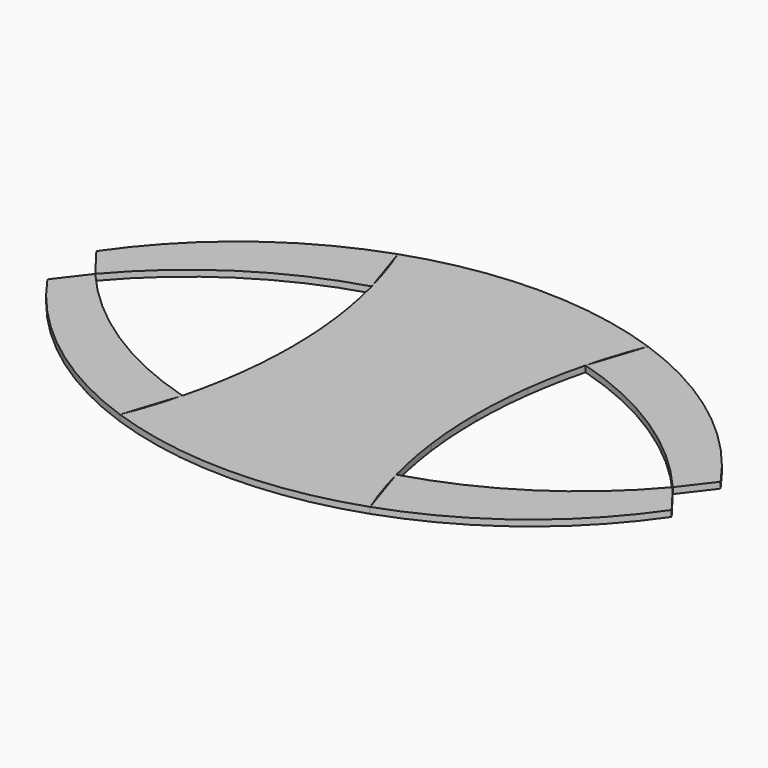
from build123d import *

# Parameters (mm, degrees)
F1_DEPTH = 10
F2_DEPTH = 10


# Not quite as in the source:
# - a feature names something its author has since deleted; it is built from what else it names


with BuildPart() as f1:
    # F0 (on Top) → F1 (new body)
    with BuildSketch(Plane.XY):
        with BuildLine():
            ThreePointArc((-424.2640687119, 50), (-448.6785937405, 74.3387267802), (-471.6990566028, 100))
            ThreePointArc((-471.6990566028, 100), (-491.4368064238, 75.4861719051), (-509.9019513593, 50))
            Line((-509.9019513593, 50), (-471.6990566028, 0))
            ThreePointArc((-471.6990566028, 0), (-448.6785937405, 25.6612732197), (-424.2640687119, 50))
        make_face()
        with BuildLine():
            ThreePointArc((-364.005494464, 100), (-394.9268616559, 124.0454076883), (-424.2640687119, 150))
            ThreePointArc((-424.2640687119, 150), (-448.6785937405, 125.6612732197), (-471.6990566028, 100))
            ThreePointArc((-471.6990566028, 100), (-448.6785937405, 74.3387267802), (-424.2640687119, 50))
            ThreePointArc((-424.2640687119, 50), (-394.9268616559, 75.9545923117), (-364.005494464, 100))
        make_face()
        with BuildLine():
            Line((-174.7028906779, 193.2780966703), (-204.3036394289, 283.7465399607))
            ThreePointArc((-204.3036394289, 283.7465399607), (-321.3197397721, 228.444533355), (-424.2640687119, 150))
            ThreePointArc((-424.2640687119, 150), (-394.9268616559, 124.0454076883), (-364.005494464, 100))
            ThreePointArc((-364.005494464, 100), (-273.362180788, 154.7730329737), (-174.7028906779, 193.2780966703))
        make_face()
    extrude(amount=F1_DEPTH)


with BuildPart() as f1b:
    # F0 (on Top) → F1, piece 2 (new body)
    with BuildSketch(Plane.XY):
        with BuildLine():
            ThreePointArc((471.6990566028, 100), (448.6785937405, 125.6612732197), (424.2640687119, 150))
            ThreePointArc((424.2640687119, 150), (394.9268616559, 124.0454076883), (364.005494464, 100))
            ThreePointArc((364.005494464, 100), (394.9268616559, 75.9545923117), (424.2640687119, 50))
            ThreePointArc((424.2640687119, 50), (448.6785937405, 74.3387267802), (471.6990566028, 100))
        make_face()
        with BuildLine():
            ThreePointArc((509.9019513593, 50), (491.4368064238, 75.4861719051), (471.6990566028, 100))
            ThreePointArc((471.6990566028, 100), (448.6785937405, 74.3387267802), (424.2640687119, 50))
            ThreePointArc((424.2640687119, 50), (448.6785937405, 25.6612732197), (471.6990566028, 0))
            Line((471.6990566028, 0), (509.9019513593, 50))
        make_face()
        with BuildLine():
            ThreePointArc((424.2640687119, 150), (321.3197397721, 228.444533355), (204.3036394289, 283.7465399607))
            Line((204.3036394289, 283.7465399607), (174.7028906779, 193.2780966703))
            ThreePointArc((174.7028906779, 193.2780966703), (273.362180788, 154.7730329737), (364.005494464, 100))
            ThreePointArc((364.005494464, 100), (394.9268616559, 124.0454076883), (424.2640687119, 150))
        make_face()
    extrude(amount=F1_DEPTH)


with BuildPart() as f1c:
    # F0 (on Top) → F1, piece 3 (new body)
    with BuildSketch(Plane.XY):
        with BuildLine():
            ThreePointArc((-424.2640687119, -50), (-448.6785937405, -25.6612732197), (-471.6990566028, 0))
            Line((-471.6990566028, 0), (-509.9019513593, -50))
            ThreePointArc((-509.9019513593, -50), (-491.4368064238, -75.4861719051), (-471.6990566028, -100))
            ThreePointArc((-471.6990566028, -100), (-448.6785937405, -74.3387267802), (-424.2640687119, -50))
        make_face()
        with BuildLine():
            ThreePointArc((-174.7028906779, -193.2780966703), (-307.9326352574, -136.3557514779), (-424.2640687119, -50))
            ThreePointArc((-424.2640687119, -50), (-448.6785937405, -74.3387267802), (-471.6990566028, -100))
            ThreePointArc((-471.6990566028, -100), (-350.2650553473, -209.7199142692), (-204.3036394289, -283.7465399607))
            Line((-204.3036394289, -283.7465399607), (-174.7028906779, -193.2780966703))
        make_face()
    extrude(amount=F1_DEPTH)


with BuildPart() as f1d:
    # F0 (on Top) → F1, piece 4 (new body)
    with BuildSketch(Plane.XY):
        with BuildLine():
            Line((509.9019513593, -50), (471.6990566028, 0))
            ThreePointArc((471.6990566028, 0), (448.6785937405, -25.6612732197), (424.2640687119, -50))
            ThreePointArc((424.2640687119, -50), (448.6785937405, -74.3387267802), (471.6990566028, -100))
            ThreePointArc((471.6990566028, -100), (491.4368064238, -75.4861719051), (509.9019513593, -50))
        make_face()
        with BuildLine():
            ThreePointArc((471.6990566028, -100), (448.6785937405, -74.3387267802), (424.2640687119, -50))
            ThreePointArc((424.2640687119, -50), (307.9326352574, -136.3557514779), (174.7028906779, -193.2780966703))
            Line((174.7028906779, -193.2780966703), (204.3036394289, -283.7465399607))
            ThreePointArc((204.3036394289, -283.7465399607), (350.2650553473, -209.7199142692), (471.6990566028, -100))
        make_face()
    extrude(amount=F1_DEPTH)


with BuildPart() as f2:
    # F0 (on Top) → F2 (new body)
    with BuildSketch(Plane.XY):
        with BuildLine():
            ThreePointArc((174.7028906779, 193.2780966703), (188.1011567973, 238.9710799865), (204.3036394289, 283.7465399607))
            ThreePointArc((204.3036394289, 283.7465399607), (0, 318.4658438426), (-204.3036394289, 283.7465399607))
            ThreePointArc((-204.3036394289, 283.7465399607), (-188.1011567973, 238.9710799865), (-174.7028906779, 193.2780966703))
            ThreePointArc((-174.7028906779, 193.2780966703), (0, 218.4658438426), (174.7028906779, 193.2780966703))
        make_face()
        with BuildLine():
            ThreePointArc((156.3238407432, 98.383536551), (164.0199022999, 146.1200685822), (174.7028906779, 193.2780966703))
            ThreePointArc((174.7028906779, 193.2780966703), (0, 218.4658438426), (-174.7028906779, 193.2780966703))
            ThreePointArc((-174.7028906779, 193.2780966703), (-164.0199022999, 146.1200685822), (-156.3238407432, 98.383536551))
            ThreePointArc((-156.3238407432, 98.383536551), (0, 118.4658438426), (156.3238407431, 98.383536551))
        make_face()
        with BuildLine():
            ThreePointArc((150, 0), (151.5825897901, 49.2932835842), (156.3238407432, 98.383536551))
            ThreePointArc((156.3238407431, 98.383536551), (0, 118.4658438426), (-156.3238407432, 98.383536551))
            ThreePointArc((-156.3238407432, 98.383536551), (-151.5825897901, 49.2932835842), (-150, 0))
            ThreePointArc((-150, 0), (0, -18.4658438426), (150, 0))
        make_face()
        with BuildLine():
            ThreePointArc((156.3238407432, -98.383536551), (151.5825897901, -49.2932835842), (150, 0))
            ThreePointArc((150, 0), (0, -18.4658438426), (-150, 0))
            ThreePointArc((-150, 0), (-151.5825897901, -49.2932835842), (-156.3238407432, -98.383536551))
            ThreePointArc((-156.3238407432, -98.383536551), (0, -118.4658438426), (156.3238407431, -98.383536551))
        make_face()
        with BuildLine():
            ThreePointArc((174.7028906779, -193.2780966703), (164.0199022999, -146.1200685822), (156.3238407432, -98.383536551))
            ThreePointArc((156.3238407431, -98.383536551), (0, -118.4658438426), (-156.3238407432, -98.383536551))
            ThreePointArc((-156.3238407432, -98.383536551), (-164.0199022999, -146.1200685822), (-174.7028906779, -193.2780966703))
            ThreePointArc((-174.7028906779, -193.2780966703), (0, -218.4658438426), (174.7028906779, -193.2780966703))
        make_face()
        with BuildLine():
            ThreePointArc((204.3036394289, -283.7465399607), (188.1011567973, -238.9710799865), (174.7028906779, -193.2780966703))
            ThreePointArc((174.7028906779, -193.2780966703), (0, -218.4658438426), (-174.7028906779, -193.2780966703))
            ThreePointArc((-174.7028906779, -193.2780966703), (-188.1011567973, -238.9710799865), (-204.3036394289, -283.7465399607))
            ThreePointArc((-204.3036394289, -283.7465399607), (0, -318.4658438426), (204.3036394289, -283.7465399607))
        make_face()
    extrude(amount=F2_DEPTH)


solid = Compound([f1.part, f1b.part, f1c.part, f1d.part, f2.part])
